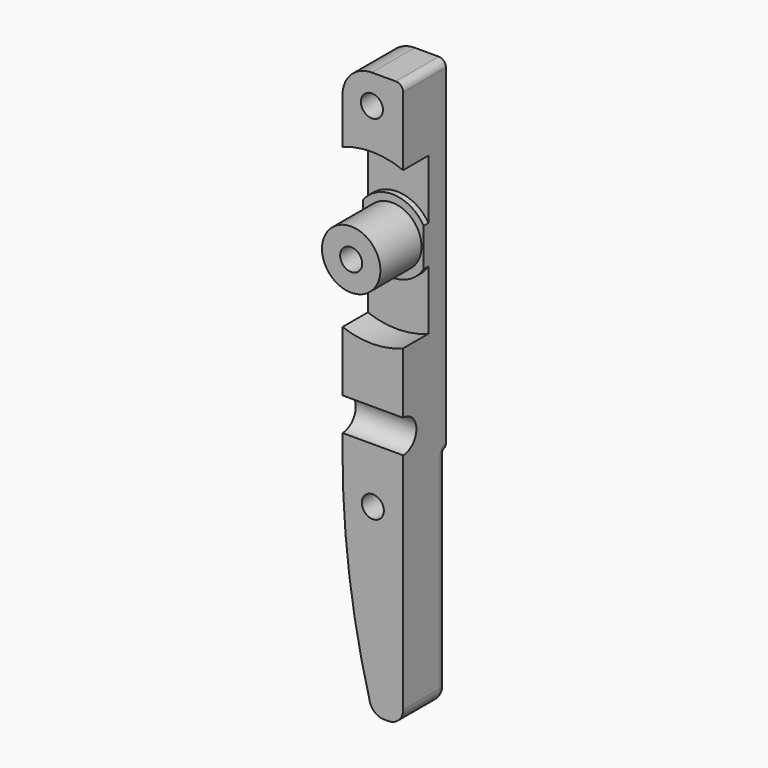
from build123d import *

# Parameters (mm, degrees)
F0_R      = 1.5
F3_DEPTH  = 3
F0_R_2    = 3.15
F5_DEPTH  = 3
F6_DEPTH  = 4.3
F7_DEPTH  = 7.8
F8_DEPTH  = 0.8
F1_R      = 2.25
F9_DEPTH  = 88
F10_DEPTH = 0.8
F12_R     = 1
F13_DEPTH = 2.4


# Not quite as in the source:
# - an extrude ends at something that could not be found from the text; its depth is read off the source's solid


with BuildPart() as f3:
    # F0 (on Front) → F3 (new body)
    with BuildSketch(Plane.XZ):
        with BuildLine():
            Line((8.25, -28), (8.25, 0))
            Line((8.25, 0), (0, 0))
            ThreePointArc((0, 0), (0.9337479911, -14.3772966716), (3.7193040011, -28.5130394045))
            ThreePointArc((3.7193040011, -28.5130394045), (4.4329720676, -29.5852568891), (5.6523820051, -30))
            Line((5.6523820051, -30), (6.25, -30))
            ThreePointArc((6.25, -30), (7.6642135624, -29.4142135624), (8.25, -28))
        make_face()
        with Locations((4.125, -5)):
            Circle(F0_R, mode=Mode.SUBTRACT)
    extrude(amount=-F3_DEPTH)

    # F4: sweep along a path in F4_path
    with BuildLine(Plane(origin=(3.7193040011, 3, -28.5130394045), x_dir=(0, 0, 1), z_dir=(0, -1, 0))) as f4_path:
        ThreePointArc((28.5130394045, 3.7193040011), (14.1357427329, 2.78555601), (0, 0))
        ThreePointArc((0, 0), (-1.0722174846, -0.7136680665), (-1.4869605955, -1.933078004))
        Line((-1.4869605955, -1.933078004), (-1.4869605955, -2.5306959989))
        ThreePointArc((-1.4869605955, -2.5306959989), (-0.9011741579, -3.9449095613), (0.5130394045, -4.5306959989))
        Line((0.5130394045, -4.5306959989), (28.5130394045, -4.5306959989))
    # F2 (on Top) → F4 (sweep, cut)
    with BuildSketch(Plane.XY):
        with BuildLine():
            ThreePointArc((7.25, 3), (7.9571067812, 2.7071067812), (8.25, 2))
            Line((8.25, 2), (8.25, 3))
            Line((8.25, 3), (7.25, 3))
        make_face()
    sweep(path=f4_path.line, mode=Mode.SUBTRACT)

    # F0 (on Front) → F5 (join, through all)
    with BuildSketch(Plane.XZ):
        with BuildLine():
            Line((8.25, 0), (8.25, 15.324121816))
            ThreePointArc((8.25, 15.324121816), (4.1356957298, 14.5011227991), (0, 15.2088288402))
            Line((0, 15.2088288402), (0, 0))
            Line((0, 0), (8.25, 0))
        make_face()
        with BuildLine():
            Line((8.25, 15.324121816), (8.25, 23.4068600115))
            ThreePointArc((8.25, 23.4068600115), (4.2412321866, 21.0070929888), (0, 22.9669528523))
            Line((0, 22.9669528523), (0, 15.2088288402))
            ThreePointArc((0, 15.2088288402), (4.1356957298, 14.5011227991), (8.25, 15.324121816))
        make_face()
        with BuildLine():
            Line((8.25, 23.4068600115), (8.25, 26))
            Line((8.25, 26), (7.95, 26))
            ThreePointArc((7.95, 26), (3.975, 22.025), (0, 26))
            Line((0, 26), (0, 22.9669528523))
            ThreePointArc((0, 22.9669528523), (4.2412321866, 21.0070929888), (8.25, 23.4068600115))
        make_face()
        with BuildLine():
            ThreePointArc((7.95, 26), (3.975, 29.975), (0, 26))
            ThreePointArc((0, 26), (3.975, 22.025), (7.95, 26))
        make_face()
        with Locations((3.975, 26)):
            Circle(F0_R, mode=Mode.SUBTRACT)
        with Locations((3.975, 26)):
            Circle(F0_R)
        with BuildLine():
            Line((8.25, 26), (8.25, 28.5931399885))
            ThreePointArc((8.25, 28.5931399885), (4.2412321866, 30.9929070112), (0, 29.0330471477))
            Line((0, 29.0330471477), (0, 26))
            ThreePointArc((0, 26), (3.975, 29.975), (7.95, 26))
            Line((7.95, 26), (8.25, 26))
        make_face()
        with BuildLine():
            Line((8.25, 28.5931399885), (8.25, 36.675878184))
            ThreePointArc((8.25, 36.675878184), (4.1356957298, 37.4988772009), (0, 36.7911711598))
            Line((0, 36.7911711598), (0, 29.0330471477))
            ThreePointArc((0, 29.0330471477), (4.2412321866, 30.9929070112), (8.25, 28.5931399885))
        make_face()
        with BuildLine():
            Line((8.25, 47), (4, 47))
            ThreePointArc((4, 47), (1.1715728753, 45.8284271247), (0, 43))
            Line((0, 43), (0, 36.7911711598))
            ThreePointArc((0, 36.7911711598), (4.1356957298, 37.4988772009), (8.25, 36.675878184))
            Line((8.25, 36.675878184), (8.25, 47))
        make_face()
        with Locations((4, 43)):
            Circle(F0_R_2, mode=Mode.SUBTRACT)
    extrude(amount=-F5_DEPTH)

    # F0 (on Front) → F6 (join)
    with BuildSketch(Plane.XZ):
        with BuildLine():
            Line((8.25, 47), (4, 47))
            ThreePointArc((4, 47), (1.1715728753, 45.8284271247), (0, 43))
            Line((0, 43), (0, 36.7911711598))
            ThreePointArc((0, 36.7911711598), (4.1356957298, 37.4988772009), (8.25, 36.675878184))
            Line((8.25, 36.675878184), (8.25, 47))
        make_face()
        with Locations((4, 43)):
            Circle(F0_R_2, mode=Mode.SUBTRACT)
        with BuildLine():
            Line((8.25, -28), (8.25, 0))
            Line((8.25, 0), (0, 0))
            ThreePointArc((0, 0), (0.9337479911, -14.3772966716), (3.7193040011, -28.5130394045))
            ThreePointArc((3.7193040011, -28.5130394045), (4.4329720676, -29.5852568891), (5.6523820051, -30))
            Line((5.6523820051, -30), (6.25, -30))
            ThreePointArc((6.25, -30), (7.6642135624, -29.4142135624), (8.25, -28))
        make_face()
        with Locations((4.125, -5)):
            Circle(F0_R, mode=Mode.SUBTRACT)
        with Locations((3.975, 26)):
            Circle(F0_R)
        with BuildLine():
            Line((8.25, 0), (8.25, 15.324121816))
            ThreePointArc((8.25, 15.324121816), (4.1356957298, 14.5011227991), (0, 15.2088288402))
            Line((0, 15.2088288402), (0, 0))
            Line((0, 0), (8.25, 0))
        make_face()
        with Locations((4, 43)):
            Circle(F0_R_2)
        with Locations((4, 43)):
            Circle(F0_R, mode=Mode.SUBTRACT)
    extrude(amount=F6_DEPTH)

    # F0 (on Front) → F7 (join)
    with BuildSketch(Plane.XZ):
        with BuildLine():
            ThreePointArc((7.95, 26), (3.975, 29.975), (0, 26))
            ThreePointArc((0, 26), (3.975, 22.025), (7.95, 26))
        make_face()
        with Locations((3.975, 26)):
            Circle(F0_R, mode=Mode.SUBTRACT)
    extrude(amount=F7_DEPTH)

    # F0 (on Front) → F8 (join)
    with BuildSketch(Plane.XZ):
        with BuildLine():
            Line((8.25, 26), (8.25, 28.5931399885))
            ThreePointArc((8.25, 28.5931399885), (4.2412321866, 30.9929070112), (0, 29.0330471477))
            Line((0, 29.0330471477), (0, 26))
            ThreePointArc((0, 26), (3.975, 29.975), (7.95, 26))
            Line((7.95, 26), (8.25, 26))
        make_face()
    extrude(amount=F8_DEPTH)

    # F1 (on Right) → F9 (cut, through all)
    with BuildSketch(Plane.YZ):
        with Locations((-4.3, 4.75)):
            Circle(F1_R)
    extrude(amount=F9_DEPTH, mode=Mode.SUBTRACT)

    # F0 (on Front) → F10 (join)
    with BuildSketch(Plane.XZ):
        with BuildLine():
            Line((8.25, 23.4068600115), (8.25, 26))
            Line((8.25, 26), (7.95, 26))
            ThreePointArc((7.95, 26), (3.975, 22.025), (0, 26))
            Line((0, 26), (0, 22.9669528523))
            ThreePointArc((0, 22.9669528523), (4.2412321866, 21.0070929888), (8.25, 23.4068600115))
        make_face()
    extrude(amount=F10_DEPTH)

    # F2 (on Top) → F11 (revolve, cut)
    with BuildSketch(Plane.XY):
        with BuildLine():
            ThreePointArc((7.25, 3), (7.9571067812, 2.7071067812), (8.25, 2))
            Line((8.25, 2), (8.25, 3))
            Line((8.25, 3), (7.25, 3))
        make_face()
    revolve(axis=Axis((7.75, 3, 0), (-1, 0, 0)), mode=Mode.SUBTRACT)

    # F12
    f12_edges = [f3.edges().sort_by_distance(p)[0] for p in [
        (8.25, -0.65, 47),
    ]]
    fillet(f12_edges, radius=F12_R)

    # F0 (on Front) → F13 (join)
    with BuildSketch(Plane.XZ):
        with Locations((4, 43)):
            Circle(F0_R_2)
        with Locations((4, 43)):
            Circle(F0_R, mode=Mode.SUBTRACT)
    extrude(amount=-F13_DEPTH)


solid = f3.part
